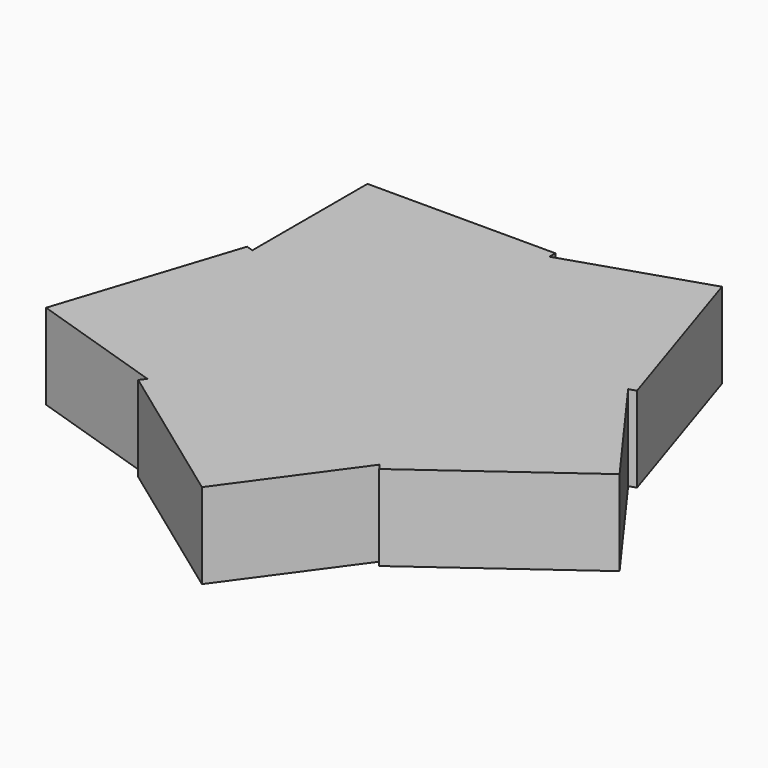
from build123d import *

# Parameters (mm, degrees)
F0_W     = 55
F0_H     = 60
F1_DEPTH = 25
F2_COUNT = 5


with BuildPart() as f1:
    # F0 (on Top) → F1 (new body)
    with BuildSketch(Plane.XY):
        with Locations((-27.5, 30)):
            Rectangle(F0_W, F0_H)
    extrude(amount=-F1_DEPTH)

    # F2: F1 ×5 about axis
    f2_axis = Axis((0, 0, -12.5), (0, 0, 1))


with BuildPart() as f1_1:
    add(f1.part)
    for i in range(1, F2_COUNT):
        add(f1.part.rotate(f2_axis, i * 360 / F2_COUNT))


solid = f1_1.part
